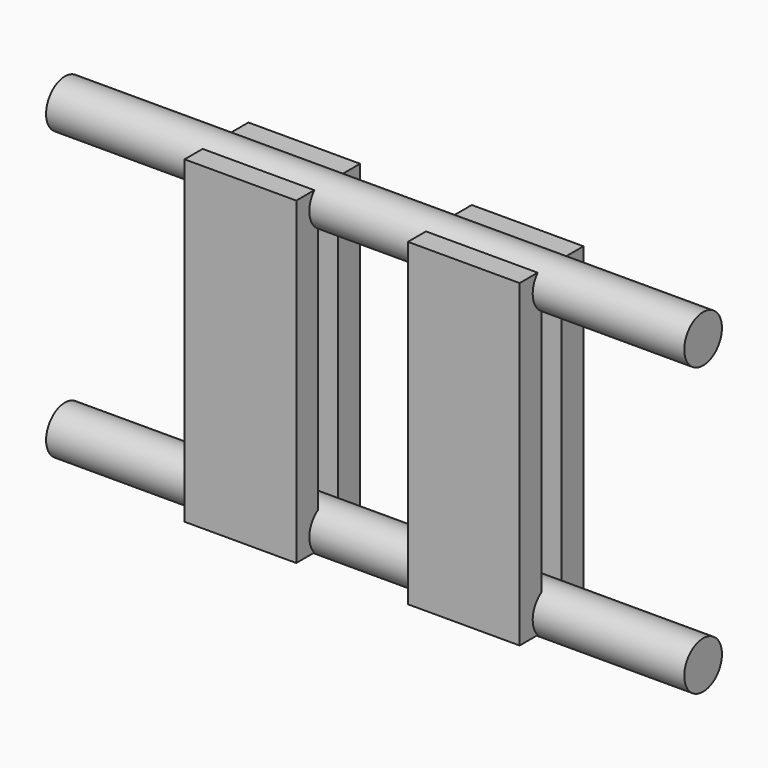
from build123d import *

# Parameters (mm, degrees)
F0_W     = 24.13
F0_H     = 4
F0_W_2   = 17.78
F1_DEPTH = 5.08
F0_H_2   = 4.35
F2_DEPTH = 50.8
F3_R     = 3.75
F3_W     = 4
F3_H     = 5.08
F4_DEPTH = 101.6
F6_DEPTH = 5.08
F7_R     = 3.75
F7_W     = 4
F7_H     = 5.08
F8_DEPTH = 101.6


with BuildPart() as f1:
    # F0 (on Top) → F1 (new body)
    with BuildSketch(Plane.XY):
        with Locations((38.735, 0)):
            Rectangle(F0_W, F0_H)
        with Locations((17.78, 0)):
            Rectangle(F0_W_2, F0_H)
        Rectangle(F0_W_2, F0_H)
        with Locations((-17.78, 0)):
            Rectangle(F0_W_2, F0_H)
        with Locations((-38.735, 0)):
            Rectangle(F0_W, F0_H)
    extrude(amount=F1_DEPTH)

    # F0 (on Top) → F2 (join)
    with BuildSketch(Plane.XY):
        with Locations((-17.78, -4.175)):
            Rectangle(F0_W_2, F0_H_2)
        with Locations((17.78, -4.175)):
            Rectangle(F0_W_2, F0_H_2)
        with Locations((-17.78, 4.175)):
            Rectangle(F0_W_2, F0_H_2)
        with Locations((17.78, 4.175)):
            Rectangle(F0_W_2, F0_H_2)
    extrude(amount=F2_DEPTH)

    # F3 (on face) → F4 (join)
    with BuildSketch(Plane(origin=(-50.8, 0, 0), x_dir=(0, -1, 0), z_dir=(-1, 0, 0))):
        with Locations((0, 2.54)):
            Circle(F3_R)
        with Locations((0, 2.54)):
            Rectangle(F3_W, F3_H, mode=Mode.SUBTRACT)
    extrude(amount=-F4_DEPTH)

    # F5 (on face) → F6 (join)
    with BuildSketch(Plane.XY.offset(50.8)):
        Polygon((-8.89, -2), (50.8, -2), (50.8, 2), (-50.8, 2), (-50.8, -2), (-26.67, -2), align=None)
    extrude(amount=-F6_DEPTH)

    # F7 (on face) → F8 (join)
    with BuildSketch(Plane(origin=(-50.8, 0, 0), x_dir=(0, -1, 0), z_dir=(-1, 0, 0))):
        with Locations((0, 48.26)):
            Circle(F7_R)
        with Locations((0, 48.26)):
            Rectangle(F7_W, F7_H, mode=Mode.SUBTRACT)
    extrude(amount=-F8_DEPTH)


solid = f1.part
